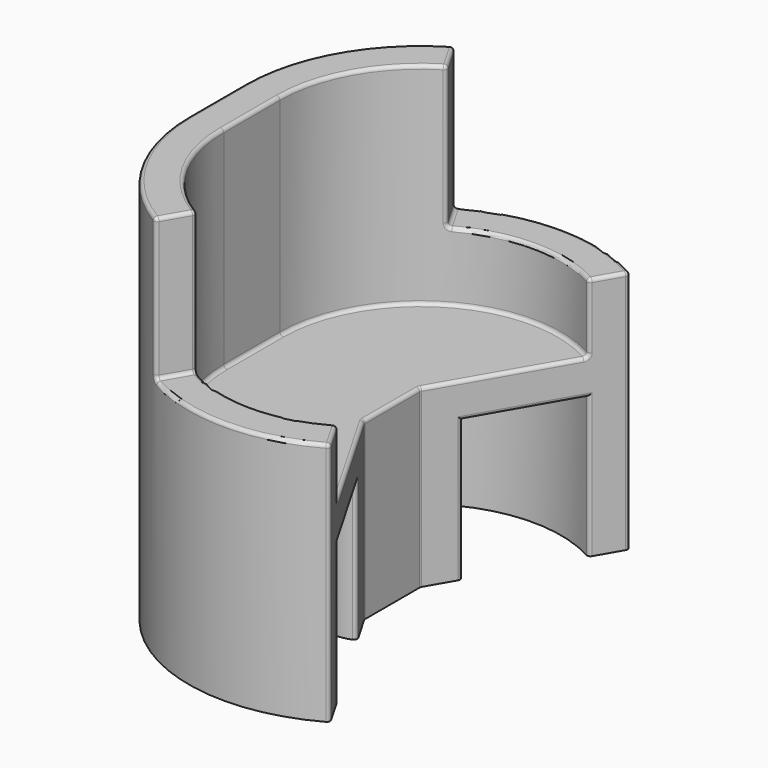
from build123d import *

# Parameters (mm, degrees)
F1_DEPTH = 10
F2_ANGLE = 120
F3_W     = 10
F3_H     = 40.4382864386
F4_ANGLE = 60
F5_R     = 1


with BuildPart() as f1:
    # F0 (on Front) → F1 (new body)
    with BuildSketch(Plane.XZ):
        Polygon((0, -50), (0, 0), (-40, 0), (-40, 60), (-50, 60), (-50, -50), (-40, -50), (-40, -10), (-10, -10), (-10, -50), align=None)
    extrude(amount=F1_DEPTH)

    # F1_face (on face) → F2 (revolve)
    with BuildSketch(Plane(origin=(-31.3157894737, -10, -4.4736842105), x_dir=(1, 0, 0), z_dir=(0, -1, 0))):
        Polygon((31.3157894737, -45.5263157895), (31.3157894737, 4.4736842105), (-8.6842105263, 4.4736842105), (-8.6842105263, 64.4736842105), (-18.6842105263, 64.4736842105), (-18.6842105263, -45.5263157895), (-8.6842105263, -45.5263157895), (-8.6842105263, -5.5263157895), (21.3157894737, -5.5263157895), (21.3157894737, -45.5263157895), align=None)
    revolve(axis=Axis((0, -10, -25), (0, 0, 1)), revolution_arc=F2_ANGLE)

    # F3 (on face) → F4 (revolve, cut)
    with BuildSketch(Plane(origin=(-4.3301270189, -2.5, 0), x_dir=(-0.5, 0.8660254038, 0), z_dir=(0.8660254038, 0.5, 0))):
        with Locations((-53.6602540378, 39.7808567807)):
            Rectangle(F3_W, F3_H)
    revolve(axis=Axis((0, -10, -25), (0, 0, -1)), revolution_arc=F4_ANGLE, mode=Mode.SUBTRACT)

    # F5
    f5_edges = [f1.edges().sort_by_distance(p)[0] for p in [
        (-34.641016, -30, 60),
        (-40, -5, 60),
        (-50, -5, 60),
        (-43.30127, -35, 60),
        (-25, -53.30127, 39.780857),
        (-20, -44.641016, 39.780857),
        (-22.5, -48.971143, 60),
        (-22.5, -48.971143, 19.561714),
        (0, -50, 19.561714),
        (0, -60, 19.561714),
        (22.5, -48.971143, 19.561714),
        (10, -27.320508, 0),
        (-20, -44.641016, 0),
        (-40, -10, 30),
        (-40, -5, 0),
        (0, -5, 0),
        (25, -53.30127, -15.219143),
        (20, -44.641016, 9.780857),
        (20, -44.641016, -30),
        (12.5, -31.650635, -10),
        (5, -18.660254, -30),
        (0, -10, -25),
    ]]
    fillet(f5_edges, radius=F5_R)

    # F6: F1 across plane


with BuildPart() as f1_1:
    add(f1.part)
    add(f1.part.mirror(Plane.XZ))


solid = f1_1.part
